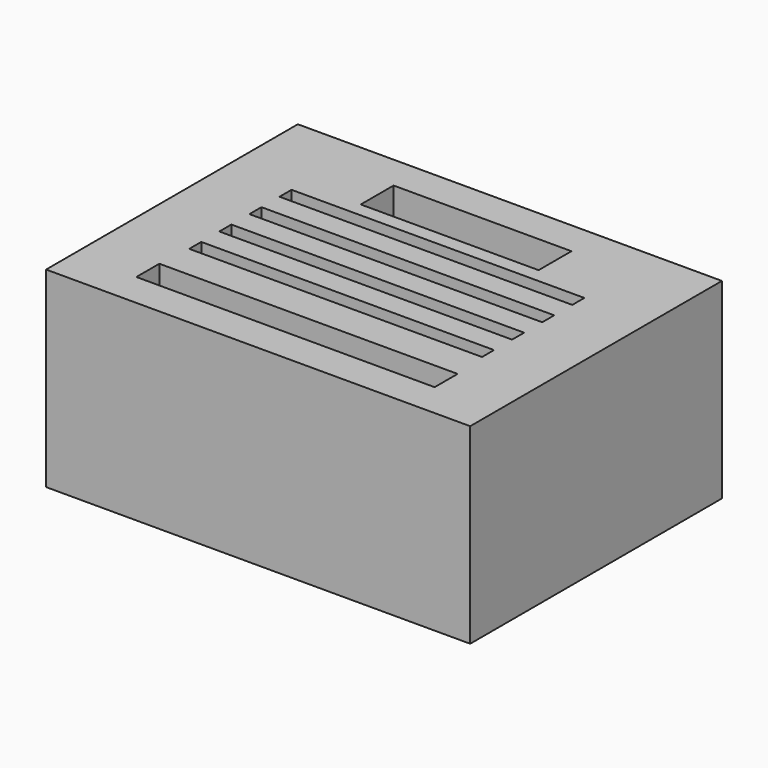
from build123d import *

# Parameters (mm, degrees)
F0_W     = 620
F0_H     = 460
F0_W_2   = 428
F0_H_2   = 22
F0_W_3   = 436
F0_H_3   = 42
F1_DEPTH = 280
F2_DEPTH = 250
F3_DEPTH = 140
F4_W     = 260
F4_H     = 60
F5_DEPTH = 40


# Not quite as in the source:
# - a feature names something its author has since deleted; it is built from what else it names


with BuildPart() as f1:
    # F0 (on Top) → F1 (new body)
    with BuildSketch(Plane.XY):
        with Locations((0.344911406, 88)):
            Rectangle(F0_W, F0_H)
        with Locations((0, 11)):
            Rectangle(F0_W_2, F0_H_2, mode=Mode.SUBTRACT)
        with Locations((0, 66)):
            Rectangle(F0_W_2, F0_H_2, mode=Mode.SUBTRACT)
        with Locations((0.344911406, -71)):
            Rectangle(F0_W_3, F0_H_3, mode=Mode.SUBTRACT)
        with Locations((0, 121)):
            Rectangle(F0_W_2, F0_H_2, mode=Mode.SUBTRACT)
        with Locations((0, 176)):
            Rectangle(F0_W_2, F0_H_2, mode=Mode.SUBTRACT)
        with Locations((0.344911406, -71)):
            Rectangle(F0_W_3, F0_H_3)
        with Locations((0, 11)):
            Rectangle(F0_W_2, F0_H_2)
        with Locations((0, 66)):
            Rectangle(F0_W_2, F0_H_2)
        with Locations((0, 121)):
            Rectangle(F0_W_2, F0_H_2)
        with Locations((0, 176)):
            Rectangle(F0_W_2, F0_H_2)
    extrude(amount=-F1_DEPTH)

    # F0 (on Top) → F2 (cut)
    with BuildSketch(Plane.XY):
        with Locations((0.344911406, -71)):
            Rectangle(F0_W_3, F0_H_3)
    extrude(amount=-F2_DEPTH, mode=Mode.SUBTRACT)

    # F0 (on Top) → F3 (cut)
    with BuildSketch(Plane.XY):
        with Locations((0, 11)):
            Rectangle(F0_W_2, F0_H_2)
        with Locations((0, 66)):
            Rectangle(F0_W_2, F0_H_2)
        with Locations((0, 121)):
            Rectangle(F0_W_2, F0_H_2)
        with Locations((0, 176)):
            Rectangle(F0_W_2, F0_H_2)
    extrude(amount=-F3_DEPTH, mode=Mode.SUBTRACT)

    # F4 (on face) → F5 (cut)
    with BuildSketch(Plane.XY):
        with Locations((0.344911406, 238)):
            Rectangle(F4_W, F4_H)
    extrude(amount=-F5_DEPTH, mode=Mode.SUBTRACT)


solid = f1.part
